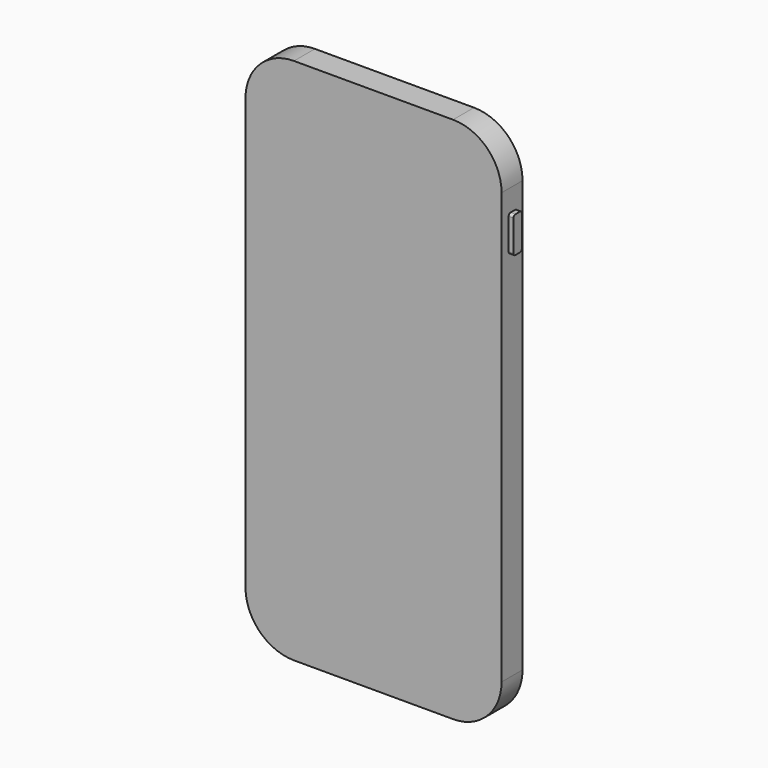
from build123d import *

# Parameters (mm, degrees)
F0_W     = 67.056
F0_H     = 138.176
F1_DEPTH = 6.858
F2_R     = 12.7
F3_R     = 12.7
F4_R     = 12.7
F5_R     = 12.7
F8_W     = 2.7374484343
F8_H     = 9.4099827111
F9_DEPTH = 1.27
F10_R    = 0.635
F11_R    = 0.635
F12_R    = 0.635
F13_R    = 0.635


# Not quite as in the source:
# - the program builds the solid bodies; features that only make, move or delete a surface that nothing else refers to are left out


with BuildPart() as f1:
    # F0 (on Front) → F1 (new body)
    with BuildSketch(Plane.XZ):
        with Locations((-33.528, 1.5209056576)):
            Rectangle(F0_W, F0_H)
    extrude(amount=F1_DEPTH)

    # F2
    f2_edges = [f1.edges().sort_by_distance(p)[0] for p in [
        (-67.056, -3.429, 70.608906),
    ]]
    fillet(f2_edges, radius=F2_R)

    # F3
    f3_edges = [f1.edges().sort_by_distance(p)[0] for p in [
        (0, -3.429, 70.608906),
    ]]
    fillet(f3_edges, radius=F3_R)

    # F4
    f4_edges = [f1.edges().sort_by_distance(p)[0] for p in [
        (-67.056, -3.429, -67.567094),
    ]]
    fillet(f4_edges, radius=F4_R)

    # F5
    f5_edges = [f1.edges().sort_by_distance(p)[0] for p in [
        (0, -3.429, -67.567094),
    ]]
    fillet(f5_edges, radius=F5_R)

    # F8 (on face) → F9 (join)
    with BuildSketch(Plane.YZ):
        with Locations((-3.1723636785, 47.4587213248)):
            Rectangle(F8_W, F8_H)
    extrude(amount=F9_DEPTH)

    # F10
    f10_edges = [f1.edges().sort_by_distance(p)[0] for p in [
        (0.635, -1.803639, 52.163713),
    ]]
    fillet(f10_edges, radius=F10_R)

    # F11
    f11_edges = [f1.edges().sort_by_distance(p)[0] for p in [
        (0.635, -1.803639, 42.75373),
    ]]
    fillet(f11_edges, radius=F11_R)

    # F12
    f12_edges = [f1.edges().sort_by_distance(p)[0] for p in [
        (0.635, -4.541088, 52.163713),
    ]]
    fillet(f12_edges, radius=F12_R)

    # F13
    f13_edges = [f1.edges().sort_by_distance(p)[0] for p in [
        (0.635, -4.541088, 42.75373),
    ]]
    fillet(f13_edges, radius=F13_R)


solid = f1.part
